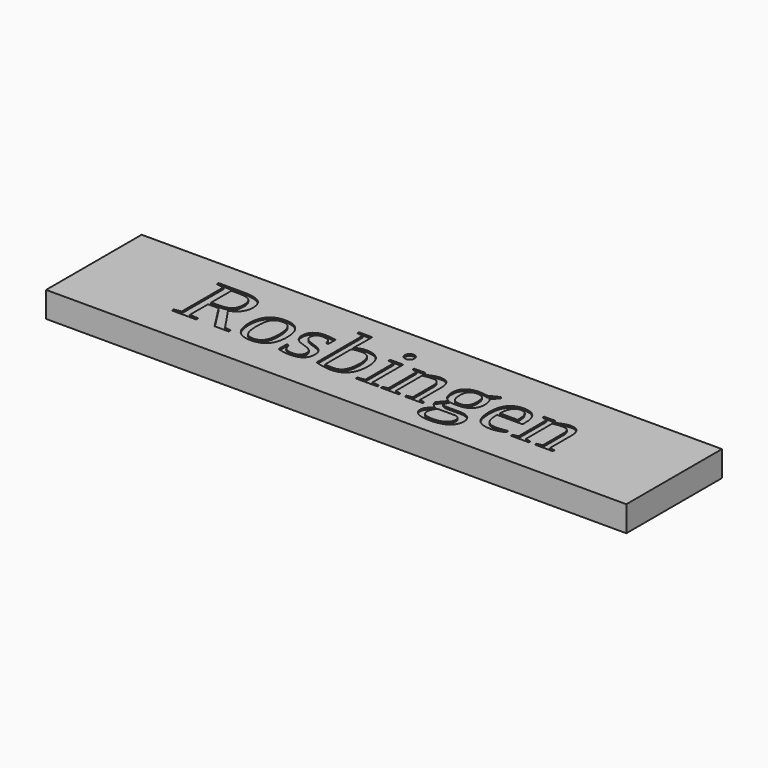
from build123d import *

# Parameters (mm, degrees)
F0_W         = 340
F0_H         = 70
F1_DEPTH     = 15
F2_TEXT_SIZE = 52.7777777778
F3_DEPTH     = 1


# Not quite as in the source:
# - Text() gives the source's letters only with a copy of the font that has no kerning and outlines rounded to 1/6400 em; it was checked with that copy


with BuildPart() as f1:
    # F0 (on Top) → F1 (new body)
    with BuildSketch(Plane.XY):
        with Locations((1.1496338993, 45.7458090895)):
            Rectangle(F0_W, F0_H)
    extrude(amount=F1_DEPTH)

    # F2 (on face) → F3 (cut)
    with BuildSketch(Plane.XY.offset(15)):
        with Locations((-112.9905570729, 30.7458090895)):
            Text('Rosbingen', F2_TEXT_SIZE, font='Tinos', text_align=(TextAlign.LEFT, TextAlign.BOTTOM))
    extrude(amount=-F3_DEPTH, mode=Mode.SUBTRACT)


solid = f1.part
